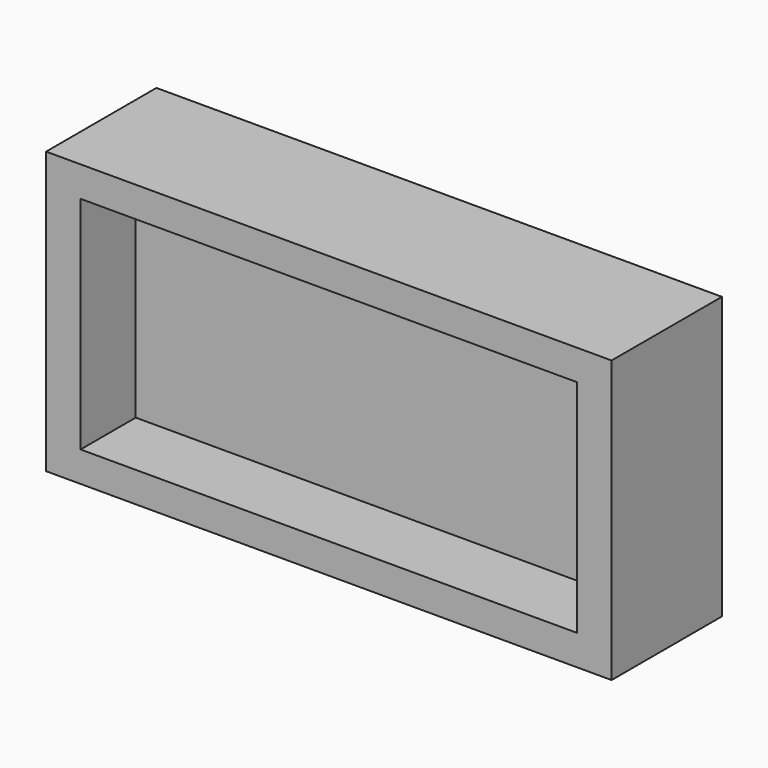
from build123d import *

# Parameters (mm, degrees)
F0_W     = 102.5
F0_H     = 51
F1_DEPTH = 25
F2_W     = 90
F2_H     = 40
F3_DEPTH = 12.5


# Not quite as in the source:
# - the program builds the solid bodies; features that only make, move or delete a surface that nothing else refers to are left out


with BuildPart() as f1:
    # F0 (on Front) → F1 (new body)
    with BuildSketch(Plane.XZ):
        Rectangle(F0_W, F0_H)
    extrude(amount=F1_DEPTH)

    # F2 (on face) → F3 (cut, symmetric)
    with BuildSketch(Plane.XZ.offset(25)):
        Rectangle(F2_W, F2_H)
    extrude(amount=F3_DEPTH, both=True, mode=Mode.SUBTRACT)


solid = f1.part
